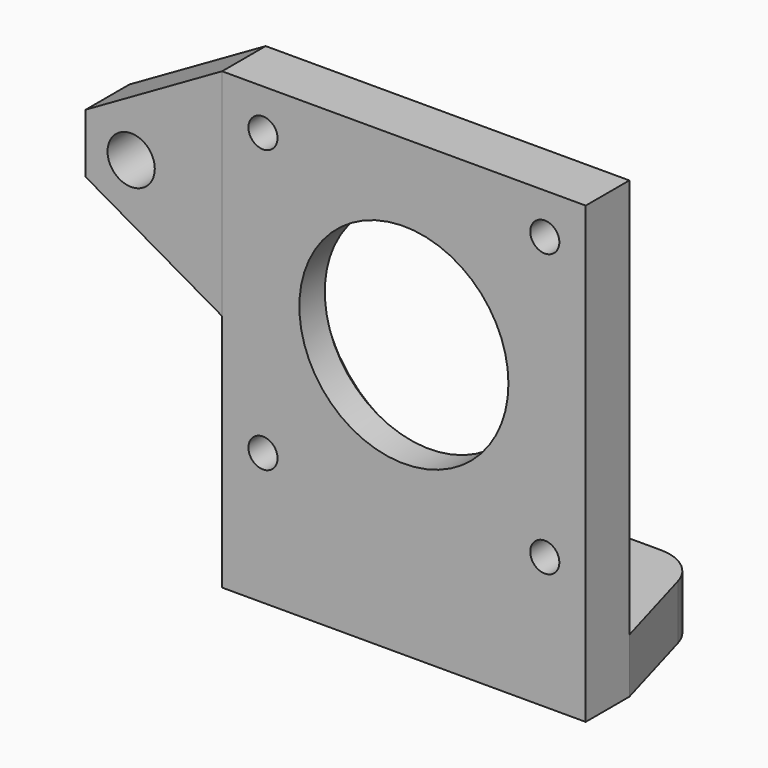
from build123d import *

# Parameters (mm, degrees)
F1_W     = 12
F1_H     = 14
F1_R     = 2.6
F2_DEPTH = 6
F3_DEPTH = 50
F4_R     = 11.5
F4_R_2   = 1.6
F5_DEPTH = 20.001
F6_R     = 2.6
F7_DEPTH = 6
F8_R     = 5
F9_SIZE  = 2.5


# Not quite as in the source:
# - a feature names something its author has since deleted; it is built from what else it names


with BuildPart() as f2:
    # F1 (on Top) → F2 (new body)
    with BuildSketch(Plane.XY):
        with Locations((-10, 30.4999971617)):
            Rectangle(F1_W, F1_H)
        with Locations((-10, 30.4999971617)):
            Circle(F1_R, mode=Mode.SUBTRACT)
        with BuildLine():
            Line((10, 33.0999971617), (10, 37.4999971617))
            Line((10, 37.4999971617), (4, 37.4999971617))
            Line((4, 37.4999971617), (4, 30.4999971617))
            Line((4, 30.4999971617), (7.4, 30.4999971617))
            ThreePointArc((7.4, 30.4999971617), (8.1615223689, 32.3384747928), (10, 33.0999971617))
        make_face()
        with BuildLine():
            Line((16, 30.4999971617), (16, 37.4999971617))
            Line((16, 37.4999971617), (10, 37.4999971617))
            Line((10, 37.4999971617), (10, 33.0999971617))
            ThreePointArc((10, 33.0999971617), (11.8384776311, 32.3384747928), (12.6, 30.4999971617))
            Line((12.6, 30.4999971617), (16, 30.4999971617))
        make_face()
        with BuildLine():
            Line((10, 23.4999971617), (16, 23.4999971617))
            Line((16, 23.4999971617), (16, 30.4999971617))
            Line((16, 30.4999971617), (12.6, 30.4999971617))
            ThreePointArc((12.6, 30.4999971617), (11.8384776311, 28.6615195306), (10, 27.8999971617))
            Line((10, 27.8999971617), (10, 23.4999971617))
        make_face()
        with BuildLine():
            Line((4, 23.4999971617), (10, 23.4999971617))
            Line((10, 23.4999971617), (10, 27.8999971617))
            ThreePointArc((10, 27.8999971617), (8.1615223689, 28.6615195306), (7.4, 30.4999971617))
            Line((7.4, 30.4999971617), (4, 30.4999971617))
            Line((4, 30.4999971617), (4, 23.4999971617))
        make_face()
        Polygon((-16, 37.4999971617), (-20, 23.4999971617), (-16, 23.4999971617), align=None)
        Polygon((-4, 37.4999971617), (-4, 23.4999971617), (4, 23.4999971617), (4, 30.4999971617), (4, 37.4999971617), align=None)
        Polygon((16, 23.4999971617), (20, 23.4999971617), (16, 37.4999971617), (16, 30.4999971617), align=None)
    extrude(amount=F2_DEPTH)

    # F1 (on Top) → F3 (join)
    with BuildSketch(Plane.XY):
        Polygon((-20, 23.4999971617), (-20, 17.4999971617), (20, 17.4999971617), (20, 23.4999971617), (16, 23.4999971617), (10, 23.4999971617), (4, 23.4999971617), (-4, 23.4999971617), (-16, 23.4999971617), align=None)
    extrude(amount=F3_DEPTH)

    # F4 (on face) → F5 (cut, through all)
    with BuildSketch(Plane.XZ.offset(-17.4999971617)):
        with Locations((0, 30)):
            Circle(F4_R)
        with Locations((-15.5, 45.5)):
            Circle(F4_R_2)
        with Locations((-15.5, 14.5)):
            Circle(F4_R_2)
        with Locations((15.5, 14.5)):
            Circle(F4_R_2)
        with Locations((15.5, 45.5)):
            Circle(F4_R_2)
    extrude(amount=-F5_DEPTH, mode=Mode.SUBTRACT)

    # F8
    f8_edges = [f2.edges().sort_by_distance(p)[0] for p in [
        (16, 37.499997, 3),
        (-16, 37.499997, 3),
    ]]
    fillet(f8_edges, radius=F8_R)

    # F9
    f9_edges = [f2.edges().sort_by_distance(p)[0] for p in [
        (-11.5, 23.499997, 30),
    ]]
    chamfer(f9_edges, length=F9_SIZE)


with BuildPart() as f7:
    # F6 (on face) → F7 (new body)
    with BuildSketch(Plane.XZ.offset(-17.4999971617)):
        Polygon((-20, 38.1438449025), (-20, 41.4031773806), (-35, 41.4031773806), (-35, 34.8845124245), (-20, 34.8845124245), align=None)
        with Locations((-30, 38.1438449025)):
            Circle(F6_R, mode=Mode.SUBTRACT)
        Polygon((-35, 41.4031773806), (-20, 41.4031773806), (-20, 50), align=None)
        Polygon((-20, 34.8845124245), (-35, 34.8845124245), (-20, 26.287689805), align=None)
    extrude(amount=-F7_DEPTH)


solid = Compound([f2.part, f7.part])
